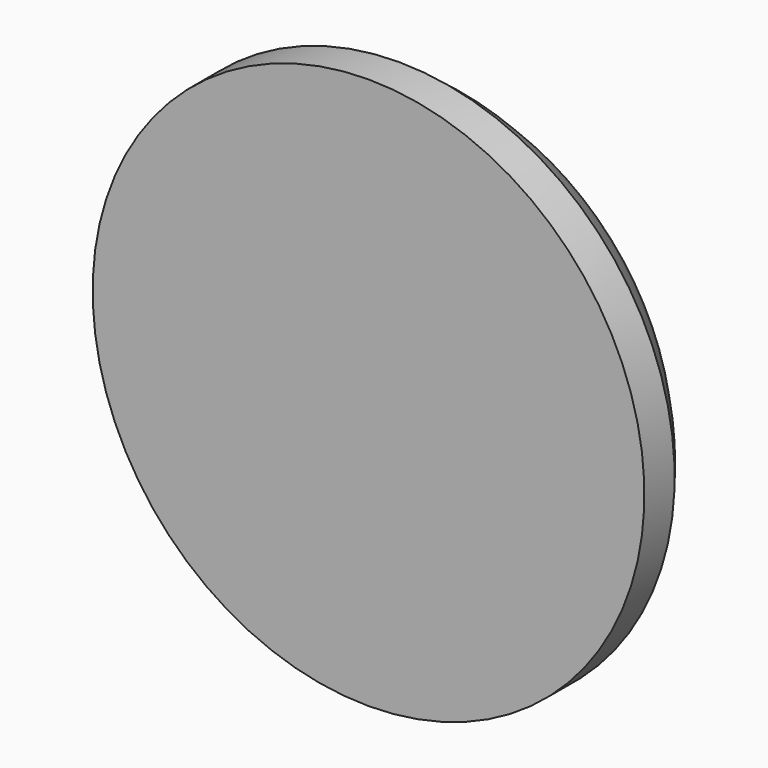
from build123d import *


# Not quite as in the source:
# - a feature names something its author has since deleted; it is built from what else it names


with BuildPart() as f1:
    # F0 (on Right) → F1 (revolve)
    with BuildSketch(Plane.YZ):
        with BuildLine():
            Line((3.75, 0), (0, 0))
            Line((0, 0), (-1, 0))
            Line((-1, 0), (-1, -7.3))
            Line((-1, -7.3), (0, -7.3))
            ThreePointArc((0, -7.3), (2.7576740388, -4.1034284446), (3.75, 0))
        make_face()
    revolve(axis=Axis((0, 1.875, 0), (0, 1, 0)))


solid = f1.part
